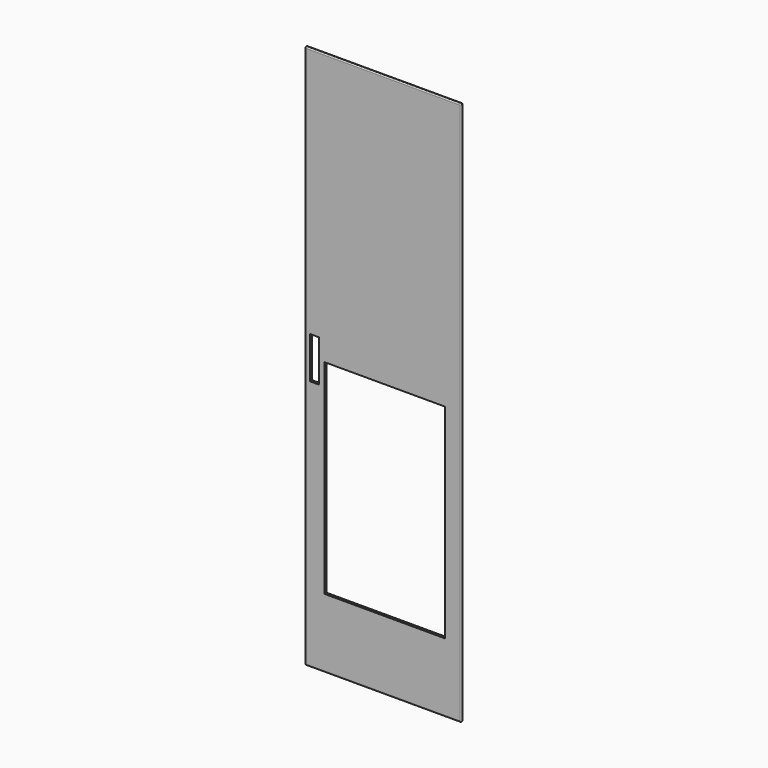
from build123d import *

# Parameters (mm, degrees)
F0_W     = 600
F0_H     = 2090
F0_W_2   = 463
F0_H_2   = 783
F0_W_3   = 35
F0_H_3   = 160
F1_DEPTH = 10
F2_R     = 4.99999


# Not quite as in the source:
# - a fillet or chamfer is up to 0.001 mm smaller than in the source, because OpenCascade refuses the exact size


with BuildPart() as f1:
    # F0 (on Front) → F1 (new body)
    with BuildSketch(Plane.XZ):
        Rectangle(F0_W, F0_H)
        with Locations((6.5, -388.5)):
            Rectangle(F0_W_2, F0_H_2, mode=Mode.SUBTRACT)
        with Locations((-262.5, 0)):
            Rectangle(F0_W_3, F0_H_3, mode=Mode.SUBTRACT)
    extrude(amount=F1_DEPTH)

    # F2 (radius 5 in the source; OpenCascade refuses exactly that, so slightly less here)
    f2_edges = [f1.edges().sort_by_distance(p)[0] for p in [
        (300, -5, 1045),
        (-300, -5, 1045),
        (-300, -5, -1045),
        (300, -5, -1045),
        (0, -10, -1045),
        (-300, -10, 0),
        (-300, 0, 0),
        (0, 0, -1045),
        (300, 0, 0),
        (300, -10, 0),
        (0, -10, 1045),
        (0, 0, 1045),
    ]]
    fillet(f2_edges, radius=F2_R)


solid = f1.part
